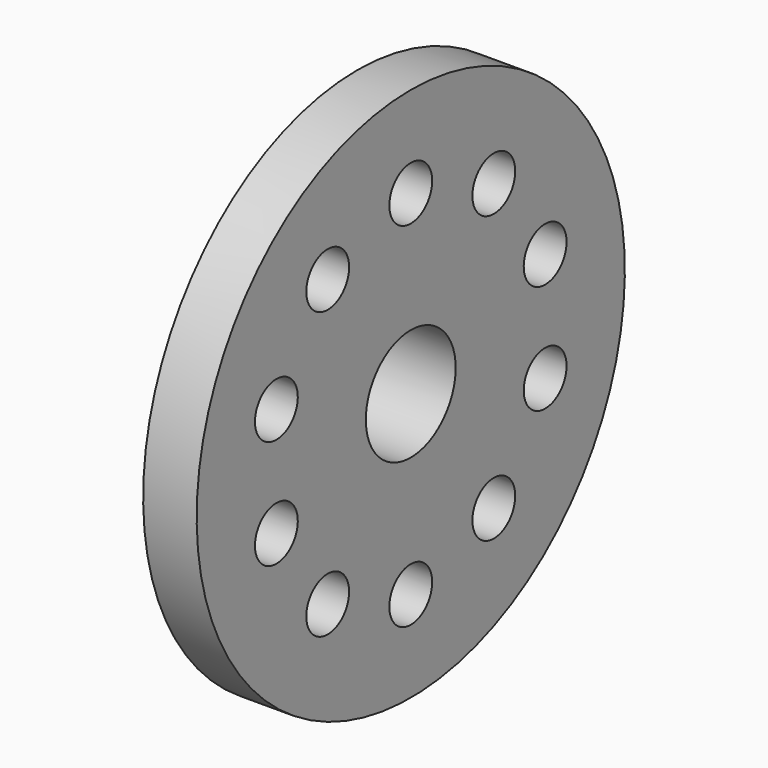
from build123d import *

# Parameters (mm, degrees)
F3_D            = 12.7
F3_COPIES_COUNT = 10


# Not quite as in the source:
# - a pattern or mirror of a feature is missing from the dataset's text; its kind, count and spacing are read off the source's solid


with BuildPart() as f1:
    # F0 (on Front) → F1 (revolve)
    with BuildSketch(Plane.XZ):
        Polygon((-25.4, 0), (0, 0), (0, 50.172699946), (-12.7, 50.172699946), (-12.7, 12.072699946), (-25.4, 12.072699946), align=None)
    revolve(axis=Axis((-12.7, 0, -13.327300054), (-1, 0, 0)))

    # F3 (through all)
    with Locations(Plane.YZ):
        with Locations((0, 28.582699946)):
            f3 = Hole(F3_D / 2)

    # F3_copies: F3 ×10 about axis
    f3_copies_axis = Axis((0, 0, -13.3273), (1, 0, 0))
    for i in range(1, F3_COPIES_COUNT):
        add(f3.rotate(f3_copies_axis, i * 360 / F3_COPIES_COUNT), mode=Mode.SUBTRACT)


solid = f1.part
